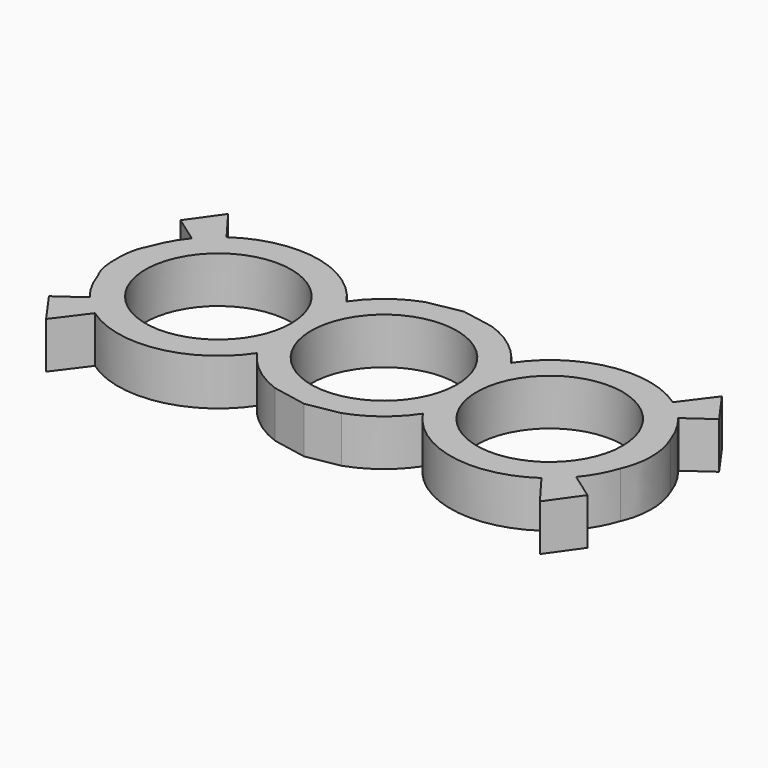
from build123d import *

# Parameters (mm, degrees)
F0_R     = 11
F1_DEPTH = 7


# Not quite as in the source:
# - a feature of the source that left no trace in its solid (it failed there, or was rolled back) is left out


with BuildPart() as f1:
    # F0 (on Top) → F1 (new body)
    with BuildSketch(Plane.XY):
        with BuildLine():
            ThreePointArc((-33.6919065778, -12.4136305481), (-22.2121981946, -14.8954900703), (-12.4070507332, -8.4300113941))
            ThreePointArc((-12.4070507332, -8.4300113941), (-9.2272824926, -11.8261260691), (-5.1598693222, -14.0845925954))
            Line((-5.1598693222, -14.0845925954), (0, -15.0684863329))
            Line((0, -15.0684863329), (4.9237644598, -14.1688582301))
            ThreePointArc((4.9237644598, -14.1688582301), (9.1941581889, -11.851896692), (12.5, -8.2915619759))
            ThreePointArc((12.5, -8.2915619759), (22.2312035836, -14.7988434658), (33.6847114379, -12.378472956))
            add(Edge.make_bspline(
                [(36.6861147035, -9.6232201138), (35.4322184653, -9.3782649416), (32.9856759013, -8.9056095075), (33.4504308992, -11.233519818), (33.6847114379, -12.378472956)],
                knots=[0.0023635799, 0.0023635799, 0.0023635799, 0.0023635799, 0.5096931431, 0.9950324973, 0.9950324973, 0.9950324973, 0.9950324973], degree=3))
            ThreePointArc((36.6861147035, -9.6232201138), (38.2829241904, -7.281044503), (39.4129405486, -4.6813041007))
            add(Edge.make_bspline(
                [(39.3532489974, 4.8612453714), (40.0640178656, 3.2496024167), (40.675386779, 0.0090485332), (40.094980448, -3.1441618112), (39.4129405486, -4.6813041007)],
                knots=[0, 0, 0, 0, 0.5048307155, 1, 1, 1, 1], degree=3))
            ThreePointArc((39.3532489974, 4.8612453714), (38.2366644679, 7.3653393625), (36.6849282767, 9.6257292672))
            add(Edge.make_bspline(
                [(33.6844640266, 12.3797240959), (33.4791642411, 11.4442056961), (33.0552816759, 9.4534774659), (35.4207112642, 9.5639432605), (36.6849282767, 9.6257292672)],
                knots=[0.0055976008, 0.0055976008, 0.0055976008, 0.0055976008, 0.4689523637, 0.9973928627, 0.9973928627, 0.9973928627, 0.9973928627], degree=3))
            ThreePointArc((33.6844640266, 12.3797240959), (22.2307373346, 14.7998328025), (12.4996432587, 8.2920997584))
            ThreePointArc((12.4996432587, 8.2920997584), (9.1939032334, 11.8520944704), (4.9237644598, 14.1688582301))
            Line((4.9237644598, 14.1688582301), (0, 15.0684863329))
            Line((0, 15.0684863329), (-5.1598693222, 14.0845925954))
            ThreePointArc((-5.1598693222, 14.0845925954), (-9.2272824926, 11.8261260691), (-12.4070507332, 8.4300113941))
            ThreePointArc((-12.4070507332, 8.4300113941), (-22.2121981946, 14.8954900703), (-33.6919065778, 12.4136305481))
            Line((-33.6919065778, 12.4136305481), (-37.2543297708, 17.1683672816))
            Line((-37.2543297708, 17.1683672816), (-40.6296290457, 12.4136305481))
            Line((-40.6296290457, 12.4136305481), (-36.703640056, 9.6266439002))
            ThreePointArc((-36.703640056, 9.6266439002), (-38.2445317988, 7.3640913066), (-39.3532489974, 4.8612453714))
            add(Edge.make_bspline(
                [(-39.3532489974, 4.8612453714), (-40.2528289587, 3.2490634103), (-40.4878486023, 0.0095823751), (-40.2812252759, -3.1446904889), (-39.4129405486, -4.6813041007)],
                knots=[0, 0, 0, 0, 0.5048307155, 1, 1, 1, 1], degree=3))
            ThreePointArc((-39.4129405486, -4.6813041007), (-38.2903364161, -7.2811002801), (-36.703640056, -9.6266439002))
            Line((-36.703640056, -9.6266439002), (-40.6296290457, -12.4136305481))
            Line((-40.6296290457, -12.4136305481), (-37.2543297708, -17.1683672816))
            Line((-37.2543297708, -17.1683672816), (-33.6919065778, -12.4136305481))
        make_face()
        with Locations((-25, 0)):
            Circle(F0_R, mode=Mode.SUBTRACT)
        with BuildLine():
            ThreePointArc((0, -11), (-11, 0), (0, 11))
            ThreePointArc((0, 11), (11, 0), (0, -11))
        make_face(mode=Mode.SUBTRACT)
        with Locations((25, 0)):
            Circle(F0_R, mode=Mode.SUBTRACT)
        with BuildLine():
            ThreePointArc((33.8754488345, -12.2437849019), (33.7803409626, -12.3114982961), (33.6847114379, -12.378472956))
            add(Edge.make_bspline(
                [(33.6847114379, -12.378472956), (33.6871093254, -12.3901916797), (33.6895079516, -12.4019111139), (33.6919065778, -12.4136305481)],
                knots=[0.9950324973, 0.9950324973, 0.9950324973, 0.9950324973, 1, 1, 1, 1], degree=3))
            Line((33.6919065778, -12.4136305481), (33.8754488345, -12.2437849019))
        make_face()
        with BuildLine():
            add(Edge.make_bspline(
                [(36.6861147035, -9.6232201138), (35.4322184653, -9.3782649416), (32.9856759013, -8.9056095075), (33.4504308992, -11.233519818), (33.6847114379, -12.378472956)],
                knots=[0.0023635799, 0.0023635799, 0.0023635799, 0.0023635799, 0.5096931431, 0.9950324973, 0.9950324973, 0.9950324973, 0.9950324973], degree=3))
            ThreePointArc((33.6847114379, -12.378472956), (33.7803409626, -12.3114982961), (33.8754488345, -12.2437849019))
            Line((33.8754488345, -12.2437849019), (33.6919065778, -12.4136305481))
            Line((33.6919065778, -12.4136305481), (37.2543297708, -17.1683672816))
            Line((37.2543297708, -17.1683672816), (40.6296290457, -12.4136305481))
            Line((40.6296290457, -12.4136305481), (36.703640056, -9.6266439002))
            Line((36.703640056, -9.6266439002), (36.6135832636, -9.7099803175))
            ThreePointArc((36.6135832636, -9.7099803175), (36.6499303523, -9.6666682398), (36.6861147035, -9.6232201138))
        make_face()
        with BuildLine():
            add(Edge.make_bspline(
                [(36.703640056, -9.6266439002), (36.6977982463, -9.6255026135), (36.6919564367, -9.6243613269), (36.6861147035, -9.6232201138)],
                knots=[0, 0, 0, 0, 0.0023635799, 0.0023635799, 0.0023635799, 0.0023635799], degree=3))
            ThreePointArc((36.6861147035, -9.6232201138), (36.6499303523, -9.6666682398), (36.6135832636, -9.7099803175))
            Line((36.6135832636, -9.7099803175), (36.703640056, -9.6266439002))
        make_face()
        with BuildLine():
            ThreePointArc((36.6176990871, 9.7061716321), (36.6513836228, 9.6660089023), (36.6849282767, 9.6257292672))
            add(Edge.make_bspline(
                [(36.6849282767, 9.6257292672), (36.6911654734, 9.6260340973), (36.6974027647, 9.6263389988), (36.703640056, 9.6266439002)],
                knots=[0.9973928627, 0.9973928627, 0.9973928627, 0.9973928627, 1, 1, 1, 1], degree=3))
            Line((36.703640056, 9.6266439002), (36.6176990871, 9.7061716321))
        make_face()
        with BuildLine():
            add(Edge.make_bspline(
                [(33.6844640266, 12.3797240959), (33.4791642411, 11.4442056961), (33.0552816759, 9.4534774659), (35.4207112642, 9.5639432605), (36.6849282767, 9.6257292672)],
                knots=[0.0055976008, 0.0055976008, 0.0055976008, 0.0055976008, 0.4689523637, 0.9973928627, 0.9973928627, 0.9973928627, 0.9973928627], degree=3))
            ThreePointArc((36.6849282767, 9.6257292672), (36.6513836228, 9.6660089023), (36.6176990871, 9.7061716321))
            Line((36.6176990871, 9.7061716321), (36.703640056, 9.6266439002))
            Line((36.703640056, 9.6266439002), (40.6296290457, 12.4136305481))
            Line((40.6296290457, 12.4136305481), (37.2543297708, 17.1683672816))
            Line((37.2543297708, 17.1683672816), (33.6919065778, 12.4136305481))
            Line((33.6919065778, 12.4136305481), (33.8702569567, 12.2485893424))
            ThreePointArc((33.8702569567, 12.2485893424), (33.777607815, 12.3145071292), (33.6844640266, 12.3797240959))
        make_face()
        with BuildLine():
            add(Edge.make_bspline(
                [(33.6919065778, 12.4136305481), (33.6894253739, 12.4023281311), (33.68694417, 12.391025714), (33.6844640266, 12.3797240959)],
                knots=[0, 0, 0, 0, 0.0055976008, 0.0055976008, 0.0055976008, 0.0055976008], degree=3))
            ThreePointArc((33.6844640266, 12.3797240959), (33.777607815, 12.3145071292), (33.8702569567, 12.2485893424))
            Line((33.8702569567, 12.2485893424), (33.6919065778, 12.4136305481))
        make_face()
    extrude(amount=F1_DEPTH)


solid = f1.part
